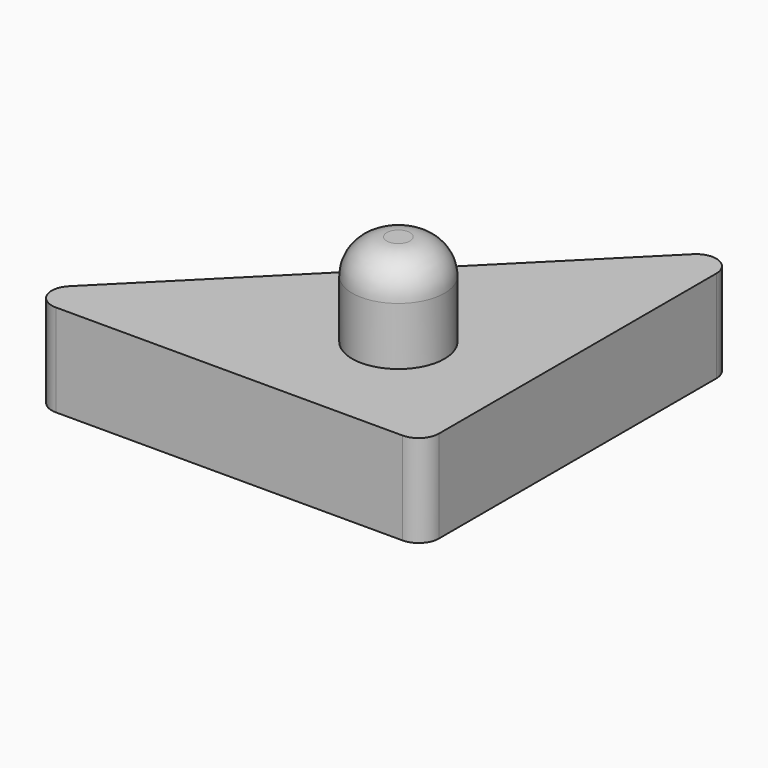
from build123d import *

# Parameters (mm, degrees)
F0_R     = 4
F1_DEPTH = 11
F2_DEPTH = 3
F3_DEPTH = 5
F4_R     = 3


# Not quite as in the source:
# - a feature names something its author has since deleted; it is built from what else it names


with BuildPart() as f1:
    # F0 (on Top) → F1 (new body)
    with BuildSketch(Plane.XY):
        with Locations((-10.5441558773, 10.5441558773)):
            Circle(F0_R)
    extrude(amount=F1_DEPTH)

    # F0 (on Top) → F2 (join)
    with BuildSketch(Plane.XY):
        with BuildLine():
            ThreePointArc((-30.0251262658, 1.75), (-30.5376893988, 0.5125631329), (-31.7751262658, 0))
            Line((-31.7751262658, 0), (-1.7499999988, 0))
            ThreePointArc((-1.7499999988, 0), (-2.9874368675, 2.9874368666), (0, 1.75))
            Line((0, 1.75), (0, 31.7751262658))
            ThreePointArc((0, 31.7751262658), (-2.4196959983, 30.1583370805), (-2.9874368799, 33.0125631201))
            Line((-2.9874368799, 33.0125631201), (-33.0125631516, 2.9874368484))
            ThreePointArc((-33.0125631516, 2.9874368484), (-31.1054302714, 3.3667891869), (-30.0251262658, 1.75))
        make_face()
        Polygon((-3, 3), (-28.7573593129, 3), (-3, 28.7573593129), align=None, mode=Mode.SUBTRACT)
        Polygon((-3, 28.7573593129), (-28.7573593129, 3), (-3, 3), align=None)
        with Locations((-10.5441558773, 10.5441558773)):
            Circle(F0_R, mode=Mode.SUBTRACT)
        with BuildLine():
            ThreePointArc((-33.0125631516, 2.9874368484), (-33.3919154427, 1.0803039812), (-31.7751262658, 0))
            ThreePointArc((-31.7751262658, 0), (-30.5376893988, 0.5125631329), (-30.0251262658, 1.75))
            ThreePointArc((-30.0251262658, 1.75), (-31.1054302714, 3.3667891869), (-33.0125631516, 2.9874368484))
        make_face()
        with BuildLine():
            ThreePointArc((0, 1.75), (-2.9874368675, 2.9874368666), (-1.7499999988, 0))
            ThreePointArc((-1.7499999988, 0), (-0.5125631325, 0.5125631334), (0, 1.75))
        make_face()
        with BuildLine():
            ThreePointArc((0, 31.7751262658), (-1.0803040017, 33.3919154512), (-2.9874368799, 33.0125631201))
            ThreePointArc((-2.9874368799, 33.0125631201), (-2.4196959983, 30.1583370805), (0, 31.7751262658))
        make_face()
    extrude(amount=F2_DEPTH)

    # F0 (on Top) → F3 (join)
    with BuildSketch(Plane.XY):
        with BuildLine():
            ThreePointArc((-30.0251262658, 1.75), (-30.5376893988, 0.5125631329), (-31.7751262658, 0))
            Line((-31.7751262658, 0), (-1.7499999988, 0))
            ThreePointArc((-1.7499999988, 0), (-2.9874368675, 2.9874368666), (0, 1.75))
            Line((0, 1.75), (0, 31.7751262658))
            ThreePointArc((0, 31.7751262658), (-2.4196959983, 30.1583370805), (-2.9874368799, 33.0125631201))
            Line((-2.9874368799, 33.0125631201), (-33.0125631516, 2.9874368484))
            ThreePointArc((-33.0125631516, 2.9874368484), (-31.1054302714, 3.3667891869), (-30.0251262658, 1.75))
        make_face()
        Polygon((-3, 3), (-28.7573593129, 3), (-3, 28.7573593129), align=None, mode=Mode.SUBTRACT)
        with BuildLine():
            ThreePointArc((0, 1.75), (-2.9874368675, 2.9874368666), (-1.7499999988, 0))
            ThreePointArc((-1.7499999988, 0), (-0.5125631325, 0.5125631334), (0, 1.75))
        make_face()
        with BuildLine():
            ThreePointArc((0, 31.7751262658), (-1.0803040017, 33.3919154512), (-2.9874368799, 33.0125631201))
            ThreePointArc((-2.9874368799, 33.0125631201), (-2.4196959983, 30.1583370805), (0, 31.7751262658))
        make_face()
        with BuildLine():
            ThreePointArc((-33.0125631516, 2.9874368484), (-33.3919154427, 1.0803039812), (-31.7751262658, 0))
            ThreePointArc((-31.7751262658, 0), (-30.5376893988, 0.5125631329), (-30.0251262658, 1.75))
            ThreePointArc((-30.0251262658, 1.75), (-31.1054302714, 3.3667891869), (-33.0125631516, 2.9874368484))
        make_face()
    extrude(amount=-F3_DEPTH)

    # F4
    f4_edges = [f1.edges().sort_by_distance(p)[0] for p in [
        (-14.544156, 10.544156, 11),
    ]]
    fillet(f4_edges, radius=F4_R)


solid = f1.part
